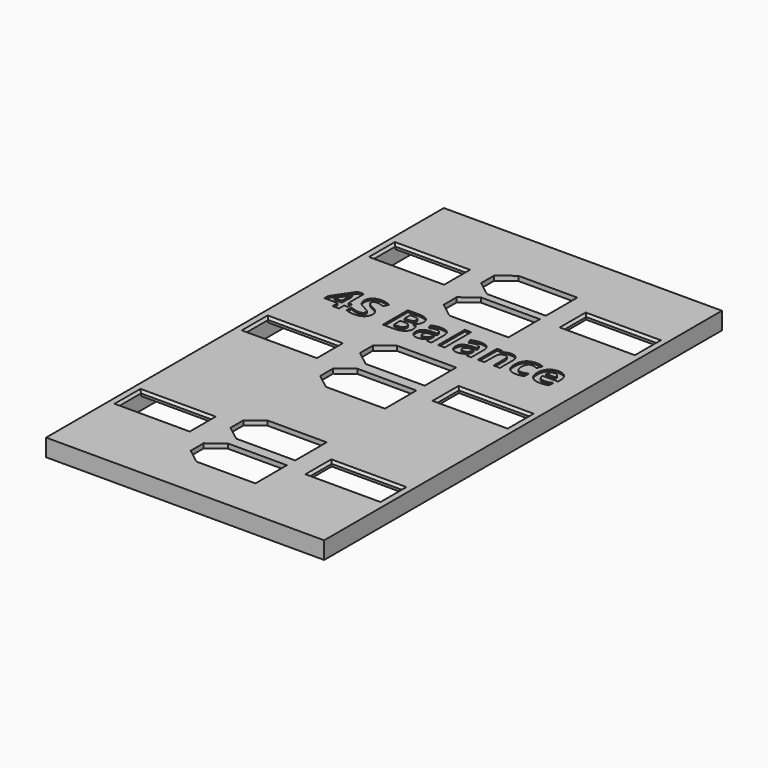
from build123d import *

# Parameters (mm, degrees)
F1_DEPTH     = 1.016
F0_W         = 61.087
F0_H         = 109.22
F2_DEPTH     = 3.81
F3_TEXT_SIZE = 9.6106890538
F4_DEPTH     = 0.381
F5_SIZE      = 0.508


# Not quite as in the source:
# - Text() gives the source's letters only with a copy of the font that has no kerning and outlines rounded to 1/6400 em; it was checked with that copy


with BuildPart() as f1:
    # F0 (on Top) → F1 (new body)
    with BuildSketch(Plane.XY):
        Polygon((28.702, 38.989), (28.702, 52.705), (-28.702, 52.705), (-28.702, 38.989), (-13.208, 38.989), (-13.208, 32.893), (-28.702, 32.893), (-28.702, 4.064), (-13.208, 4.064), (-13.208, -2.032), (-28.702, -2.032), (-28.702, -30.861), (-13.208, -30.861), (-13.208, -36.957), (-28.702, -36.957), (-28.702, -52.705), (28.702, -52.705), (28.702, -36.957), (13.208, -36.957), (13.208, -30.861), (28.702, -30.861), (28.702, -2.032), (13.208, -2.032), (13.208, 4.064), (28.702, 4.064), (28.702, 32.893), (13.208, 32.893), (13.208, 38.989), align=None)
        Polygon((-4.826, -36.83), (8.128, -36.83), (8.128, -45.466), (-4.826, -45.466), (-8.128, -45.466), (-8.128, -42.926), (-8.128, -39.37), (-8.128, -36.83), align=None, mode=Mode.SUBTRACT)
        Polygon((8.128, -25.908), (8.128, -34.544), (-4.826, -34.544), (-8.128, -34.544), (-8.128, -32.004), (-8.128, -28.448), (-8.128, -25.908), (-4.826, -25.908), align=None, mode=Mode.SUBTRACT)
        Polygon((8.128, -1.27), (8.128, -9.906), (-4.826, -9.906), (-8.128, -9.906), (-8.128, -7.366), (-8.128, -3.81), (-8.128, -1.27), (-4.826, -1.27), align=None, mode=Mode.SUBTRACT)
        Polygon((8.128, 9.652), (8.128, 1.016), (-4.826, 1.016), (-8.128, 1.016), (-8.128, 3.556), (-8.128, 7.112), (-8.128, 9.652), (-4.826, 9.652), align=None, mode=Mode.SUBTRACT)
        Polygon((8.128, 32.639), (8.128, 24.003), (-4.826, 24.003), (-8.128, 24.003), (-8.128, 26.543), (-8.128, 30.099), (-8.128, 32.639), (-4.826, 32.639), align=None, mode=Mode.SUBTRACT)
        Polygon((8.128, 42.926), (8.128, 34.29), (-4.826, 34.29), (-8.128, 34.29), (-8.128, 36.83), (-8.128, 40.386), (-8.128, 42.926), (-4.826, 42.926), align=None, mode=Mode.SUBTRACT)
        Polygon((-8.128, -45.466), (-4.826, -45.466), (-8.128, -42.926), align=None)
        Polygon((-8.128, -39.37), (-4.826, -36.83), (-8.128, -36.83), align=None)
        Polygon((-8.128, -34.544), (-4.826, -34.544), (-8.128, -32.004), align=None)
        Polygon((-8.128, -28.448), (-4.826, -25.908), (-8.128, -25.908), align=None)
        Polygon((-8.128, -9.906), (-4.826, -9.906), (-8.128, -7.366), align=None)
        Polygon((-8.128, -3.81), (-4.826, -1.27), (-8.128, -1.27), align=None)
        Polygon((-8.128, 1.016), (-4.826, 1.016), (-8.128, 3.556), align=None)
        Polygon((-8.128, 7.112), (-4.826, 9.652), (-8.128, 9.652), align=None)
        Polygon((-8.128, 24.003), (-4.826, 24.003), (-8.128, 26.543), align=None)
        Polygon((-8.128, 30.099), (-4.826, 32.639), (-8.128, 32.639), align=None)
        Polygon((-8.128, 34.29), (-4.826, 34.29), (-8.128, 36.83), align=None)
        Polygon((-8.128, 40.386), (-4.826, 42.926), (-8.128, 42.926), align=None)
    extrude(amount=-F1_DEPTH)

    # F0 (on Top) → F2 (join)
    with BuildSketch(Plane.XY):
        Rectangle(F0_W, F0_H)
        Polygon((-28.702, 52.705), (28.702, 52.705), (28.702, 38.989), (28.702, 32.893), (28.702, 4.064), (28.702, -2.032), (28.702, -30.861), (28.702, -36.957), (28.702, -52.705), (-28.702, -52.705), (-28.702, -36.957), (-28.702, -30.861), (-28.702, -2.032), (-28.702, 4.064), (-28.702, 32.893), (-28.702, 38.989), align=None, mode=Mode.SUBTRACT)
    extrude(amount=-F2_DEPTH)

    # F3 (on face) → F4 (cut)
    with BuildSketch(Plane.XY):
        with Locations((-25.781, 14.2352607664)):
            Text('4S Balance', F3_TEXT_SIZE, font='Open Sans', font_style=FontStyle.BOLD, text_align=(TextAlign.LEFT, TextAlign.BOTTOM))
    extrude(amount=-F4_DEPTH, mode=Mode.SUBTRACT)

    # F5
    f5_edges = [f1.edges().sort_by_distance(p)[0] for p in [
        (20.955, 4.064, 0),
        (13.208, 1.016, 0),
        (20.955, -2.032, 0),
        (28.702, 1.016, 0),
        (20.955, 32.893, 0),
        (20.955, 38.989, 0),
        (13.208, 35.941, 0),
        (28.702, 35.941, 0),
        (20.955, -30.861, 0),
        (20.955, -36.957, 0),
        (13.208, -33.909, 0),
        (28.702, -33.909, 0),
        (-20.955, -36.957, 0),
        (-20.955, -30.861, 0),
        (-13.208, -33.909, 0),
        (-28.702, -33.909, 0),
        (-20.955, -2.032, 0),
        (-20.955, 4.064, 0),
        (-13.208, 1.016, 0),
        (-28.702, 1.016, 0),
        (-20.955, 32.893, 0),
        (-20.955, 38.989, 0),
        (-13.208, 35.941, 0),
        (-28.702, 35.941, 0),
    ]]
    chamfer(f5_edges, length=F5_SIZE)


solid = f1.part
